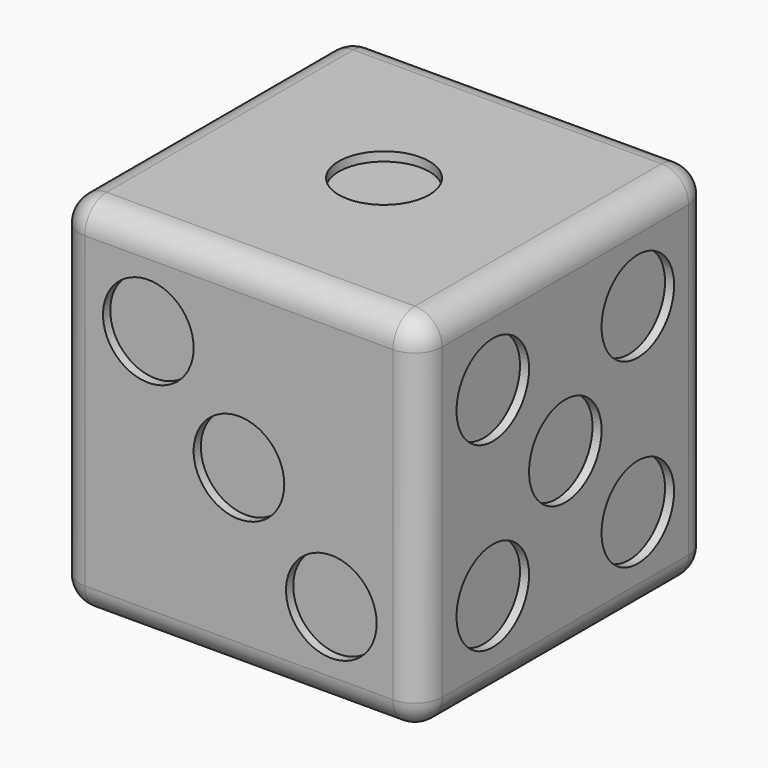
from build123d import *

# Parameters (mm, degrees)
F0_W      = 40
F0_H      = 40
F1_DEPTH  = 40
F2_R      = 5
F3_DEPTH  = 5
F4_R      = 5
F5_DEPTH  = 5
F6_DEPTH  = 4
F7_DEPTH  = 4
F8_R      = 5
F9_DEPTH  = 5
F10_DEPTH = 4
F11_R     = 5
F12_DEPTH = 5
F13_DEPTH = 4
F14_R     = 5
F15_DEPTH = 5
F16_DEPTH = 3
F17_DEPTH = 4
F18_DEPTH = 2
F19_R     = 5
F20_DEPTH = 3
F21_DEPTH = 2
F22_R     = 3


# Not quite as in the source:
# - a feature names something its author has since deleted; it is built from what else it names


with BuildPart() as f1:
    # F0 (on Top) → F1 (new body)
    with BuildSketch(Plane.XY):
        Rectangle(F0_W, F0_H)
    extrude(amount=F1_DEPTH)

    # F2 (on face) → F3 (cut)
    with BuildSketch(Plane.XY.offset(40)):
        Circle(F2_R)
    extrude(amount=-F3_DEPTH, mode=Mode.SUBTRACT)

    # F4 (on face) → F5 (cut)
    with BuildSketch(Plane.YZ.offset(20)):
        with Locations((-10, 30)):
            Circle(F4_R)
        with Locations((0, 20)):
            Circle(F4_R)
        with Locations((10, 30)):
            Circle(F4_R)
        with Locations((10, 10)):
            Circle(F4_R)
        with Locations((-10, 10)):
            Circle(F4_R)
    extrude(amount=-F5_DEPTH, mode=Mode.SUBTRACT)


with BuildPart() as f6:
    # F6 (new): a face of the model
    f6_faces = [f1.part.faces().sort_by_distance(p)[0] for p in [
        (15, -10, 30),
    ]]
    extrude(f6_faces, amount=F6_DEPTH)


with BuildPart() as f6b:
    # F6#2 (new): a face of the model
    f6_2_faces = [f1.part.faces().sort_by_distance(p)[0] for p in [
        (15, 10, 30),
    ]]
    extrude(f6_2_faces, amount=F6_DEPTH)


with BuildPart() as f6c:
    # F6#3 (new): a face of the model
    f6_3_faces = [f1.part.faces().sort_by_distance(p)[0] for p in [
        (15, 0, 20),
    ]]
    extrude(f6_3_faces, amount=F6_DEPTH)


with BuildPart() as f6d:
    # F6#4 (new): a face of the model
    f6_4_faces = [f1.part.faces().sort_by_distance(p)[0] for p in [
        (15, -10, 10),
    ]]
    extrude(f6_4_faces, amount=F6_DEPTH)


with BuildPart() as f6e:
    # F6#5 (new): a face of the model
    f6_5_faces = [f1.part.faces().sort_by_distance(p)[0] for p in [
        (15, 10, 10),
    ]]
    extrude(f6_5_faces, amount=F6_DEPTH)


with BuildPart() as f7:
    # F7 (new): a face of the model
    f7_faces = [f1.part.faces().sort_by_distance(p)[0] for p in [
        (0, 0, 35),
    ]]
    extrude(f7_faces, amount=F7_DEPTH)


with BuildPart() as f1_1:
    add(f1.part)

    # F8 (on face) → F9 (cut)
    with BuildSketch(Plane(origin=(0, 0, 0), x_dir=(1, 0, 0), z_dir=(0, 0, -1))):
        with Locations((-9, 11)):
            Circle(F8_R)
        with Locations((-9, 0)):
            Circle(F8_R)
        with Locations((-9, -11)):
            Circle(F8_R)
        with Locations((9, -11)):
            Circle(F8_R)
        with Locations((9, 0)):
            Circle(F8_R)
        with Locations((9, 11)):
            Circle(F8_R)
    extrude(amount=-F9_DEPTH, mode=Mode.SUBTRACT)


with BuildPart() as f10:
    # F10 (new): a face of the model
    f10_faces = [f1_1.part.faces().sort_by_distance(p)[0] for p in [
        (-9, -11, 5),
    ]]
    extrude(f10_faces, amount=F10_DEPTH)


with BuildPart() as f10b:
    # F10#2 (new): a face of the model
    f10_2_faces = [f1_1.part.faces().sort_by_distance(p)[0] for p in [
        (-9, 0, 5),
    ]]
    extrude(f10_2_faces, amount=F10_DEPTH)


with BuildPart() as f10c:
    # F10#3 (new): a face of the model
    f10_3_faces = [f1_1.part.faces().sort_by_distance(p)[0] for p in [
        (-9, 11, 5),
    ]]
    extrude(f10_3_faces, amount=F10_DEPTH)


with BuildPart() as f10d:
    # F10#4 (new): a face of the model
    f10_4_faces = [f1_1.part.faces().sort_by_distance(p)[0] for p in [
        (9, 11, 5),
    ]]
    extrude(f10_4_faces, amount=F10_DEPTH)


with BuildPart() as f10e:
    # F10#5 (new): a face of the model
    f10_5_faces = [f1_1.part.faces().sort_by_distance(p)[0] for p in [
        (9, 0, 5),
    ]]
    extrude(f10_5_faces, amount=F10_DEPTH)


with BuildPart() as f10f:
    # F10#6 (new): a face of the model
    f10_6_faces = [f1_1.part.faces().sort_by_distance(p)[0] for p in [
        (9, -11, 5),
    ]]
    extrude(f10_6_faces, amount=F10_DEPTH)


with BuildPart() as f1_2:
    add(f1_1.part)

    # F11 (on face) → F12 (cut)
    with BuildSketch(Plane(origin=(-20, 0, 0), x_dir=(0, -1, 0), z_dir=(-1, 0, 0))):
        with Locations((-7.2720779386, 27.2720779386)):
            Circle(F11_R)
        with Locations((7.2720779386, 12.7279220614)):
            Circle(F11_R)
    extrude(amount=-F12_DEPTH, mode=Mode.SUBTRACT)


with BuildPart() as f13:
    # F13 (new): a face of the model
    f13_faces = [f1_2.part.faces().sort_by_distance(p)[0] for p in [
        (-15, 7.2720779386, 27.2720779386),
    ]]
    extrude(f13_faces, amount=F13_DEPTH)


with BuildPart() as f13b:
    # F13#2 (new): a face of the model
    f13_2_faces = [f1_2.part.faces().sort_by_distance(p)[0] for p in [
        (-15, -7.2720779386, 12.7279220614),
    ]]
    extrude(f13_2_faces, amount=F13_DEPTH)


with BuildPart() as f1_3:
    add(f1_2.part)

    # F14 (on face) → F15 (cut)
    with BuildSketch(Plane.XZ.offset(20)):
        with Locations((-9.9999191238, 29.9999191238)):
            Circle(F14_R)
        with Locations((-1.50242e-05, 20.0000150242)):
            Circle(F14_R)
    extrude(amount=-F15_DEPTH, mode=Mode.SUBTRACT)

    # F14 (on face) → F16 (cut)
    with BuildSketch(Plane.XZ.offset(20)):
        with Locations((10.1908079062, 9.8091920938)):
            Circle(F14_R)
    extrude(amount=-F16_DEPTH, mode=Mode.SUBTRACT)


with BuildPart() as f17:
    # F17 (new): a face of the model
    f17_faces = [f1_3.part.faces().sort_by_distance(p)[0] for p in [
        (-9.9999191238, -15, 29.9999191238),
    ]]
    extrude(f17_faces, amount=F17_DEPTH)


with BuildPart() as f17b:
    # F17#2 (new): a face of the model
    f17_2_faces = [f1_3.part.faces().sort_by_distance(p)[0] for p in [
        (-1.50242e-05, -15, 20.0000150242),
    ]]
    extrude(f17_2_faces, amount=F17_DEPTH)


with BuildPart() as f18:
    # F18 (new): a face of the model
    f18_faces = [f1_3.part.faces().sort_by_distance(p)[0] for p in [
        (10.1908079062, -17, 9.8091920938),
    ]]
    extrude(f18_faces, amount=F18_DEPTH)


with BuildPart() as f1_4:
    add(f1_3.part)

    # F19 (on face) → F20 (cut)
    with BuildSketch(Plane(origin=(0, 20, 0), x_dir=(-1, 0, 0), z_dir=(0, 1, 0))):
        with Locations((-10, 30)):
            Circle(F19_R)
        with Locations((10, 30)):
            Circle(F19_R)
        with Locations((10, 10)):
            Circle(F19_R)
        with Locations((-10, 10)):
            Circle(F19_R)
    extrude(amount=-F20_DEPTH, mode=Mode.SUBTRACT)


with BuildPart() as f21:
    # F21 (new): a face of the model
    f21_faces = [f1_4.part.faces().sort_by_distance(p)[0] for p in [
        (10, 17, 30),
    ]]
    extrude(f21_faces, amount=F21_DEPTH)


with BuildPart() as f21b:
    # F21#2 (new): a face of the model
    f21_2_faces = [f1_4.part.faces().sort_by_distance(p)[0] for p in [
        (-10, 17, 30),
    ]]
    extrude(f21_2_faces, amount=F21_DEPTH)


with BuildPart() as f21c:
    # F21#3 (new): a face of the model
    f21_3_faces = [f1_4.part.faces().sort_by_distance(p)[0] for p in [
        (-10, 17, 10),
    ]]
    extrude(f21_3_faces, amount=F21_DEPTH)


with BuildPart() as f21d:
    # F21#4 (new): a face of the model
    f21_4_faces = [f1_4.part.faces().sort_by_distance(p)[0] for p in [
        (10, 17, 10),
    ]]
    extrude(f21_4_faces, amount=F21_DEPTH)


with BuildPart() as f1_5:
    add(f1_4.part)

    # F22
    f22_edges = [f1_5.edges().sort_by_distance(p)[0] for p in [
        (-20, 0, 40),
        (0, 20, 40),
        (0, -20, 40),
        (-20, -20, 20),
        (20, 0, 40),
        (20, -20, 20),
        (20, 20, 20),
        (-20, 20, 20),
        (-20, 0, 0),
        (0, 20, 0),
        (0, -20, 0),
        (20, 0, 0),
    ]]
    fillet(f22_edges, radius=F22_R)


solid = Compound([f6.part, f6b.part, f6c.part, f6d.part, f6e.part, f7.part, f10.part, f10b.part, f10c.part, f10d.part, f10e.part, f10f.part, f13.part, f13b.part, f17.part, f17b.part, f18.part, f21.part, f21b.part, f21c.part, f21d.part, f1_5.part])
